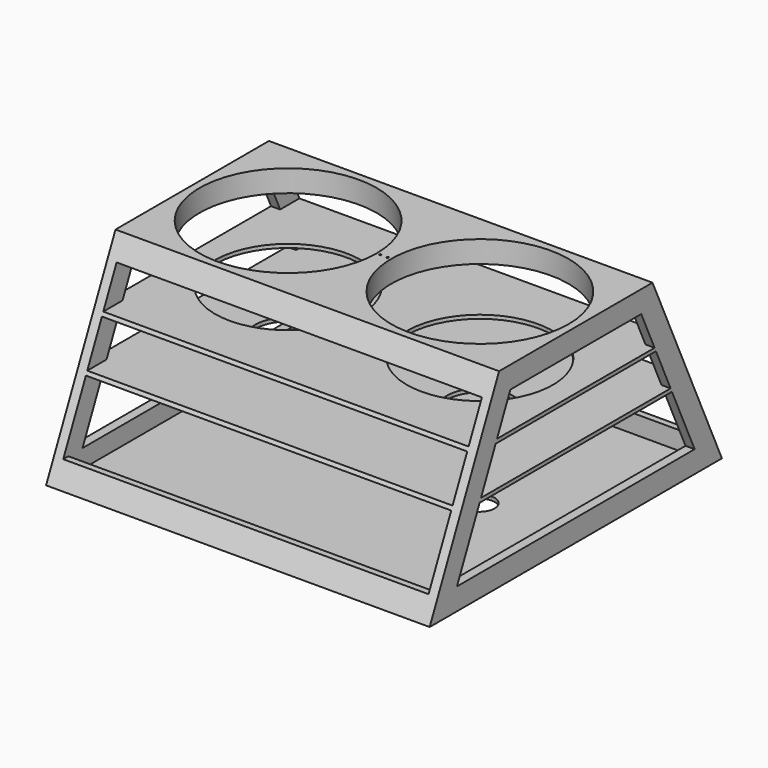
from build123d import *

# Parameters (mm, degrees)
F0_W      = 666.75
F0_H      = 635
F1_DEPTH  = 165.1
F4_W      = 333.375
F4_H      = 69.85
F5_DEPTH  = 666.751
F6_W      = 635
F6_H      = 63.5
F6_H_2    = 107.95
F6_H_3    = 69.85
F7_DEPTH  = 330.2
F9_DEPTH  = 38.1
F11_DEPTH = 25.4
F13_DEPTH = 25.4
F14_W     = 635
F14_H     = 577.849984169
F15_DEPTH = 31.75
F17_DEPTH = 25.4
F19_D     = 3.175
F19_DEPTH = 38.1
F19_TIP   = 0.9538662327


with BuildPart() as f1:
    # F0 (on Top) → F1 (new body, symmetric)
    with BuildSketch(Plane.XY):
        Rectangle(F0_W, F0_H)
    extrude(amount=F1_DEPTH, both=True)

    # F4 (on face) → F5 (cut, through all)
    with BuildSketch(Plane.YZ.offset(333.375)):
        Polygon((0, 127), (-142.2031428718, 127), (-166.6875, 73.3921443929), (-166.6875, 63.5), (166.6875, 63.5), (166.6875, 73.3921443929), (142.2031428718, 127), align=None)
        Polygon((-166.6875, 63.5), (-166.6875, 73.3921443929), (-171.2055467179, 63.5), align=None)
        Polygon((171.2055467179, 63.5), (166.6875, 73.3921443929), (166.6875, 63.5), align=None)
        Polygon((174.1057871025, 57.15), (166.6875, 57.15), (166.6875, -12.7), (206.0084313333, -12.7), align=None)
        with Locations((0, 22.225)):
            Rectangle(F4_W, F4_H)
        Polygon((-166.6875, -12.7), (-166.6875, 57.15), (-174.1057871025, 57.15), (-206.0084313333, -12.7), align=None)
        Polygon((-208.9086717179, -19.05), (-258.2127582564, -127), (-166.6875, -127), (-166.6875, -19.05), align=None)
        Polygon((-166.6875, -19.05), (-166.6875, -127), (0, -127), (166.6875, -127), (166.6875, -19.05), align=None)
        Polygon((166.6875, -19.05), (166.6875, -127), (258.2127582564, -127), (208.9086717179, -19.05), align=None)
        Polygon((317.5, 165.1), (166.6875, 165.1), (184.0889423077, 127), (213.0913461538, 63.5), (317.5, -165.1), align=None)
        Polygon((-184.0889423077, 127), (-166.6875, 165.1), (-317.5, 165.1), (-317.5, -165.1), (-213.0913461538, 63.5), align=None)
    extrude(amount=-F5_DEPTH, mode=Mode.SUBTRACT)

    # F6 (on Front) → F7 (cut, symmetric)
    with BuildSketch(Plane.XZ):
        with Locations((0, 95.25)):
            Rectangle(F6_W, F6_H)
        with Locations((0, -73.025)):
            Rectangle(F6_W, F6_H_2)
        with Locations((0, 22.225)):
            Rectangle(F6_W, F6_H_3)
    extrude(amount=F7_DEPTH, both=True, mode=Mode.SUBTRACT)

    # F3 (on face) + F8 (on face) → F9 (cut)
    with BuildSketch(Plane.XY.offset(165.1)):
        with BuildLine():
            ThreePointArc((-166.6875, 153.9875), (-320.675, 0), (-166.6875, -153.9875))
            Line((-166.6875, -153.9875), (-166.6875, 153.9875))
        make_face()
        with BuildLine():
            Line((-166.6875, 153.9875), (-166.6875, -153.9875))
            ThreePointArc((-166.6875, -153.9875), (-57.801894532, -108.885605468), (-12.7, 0))
            ThreePointArc((-12.7, 0), (-57.801894532, 108.885605468), (-166.6875, 153.9875))
        make_face()
        with BuildLine():
            ThreePointArc((166.6875, 153.9875), (12.7, 0), (166.6875, -153.9875))
            Line((166.6875, -153.9875), (166.6875, 153.9875))
        make_face()
    with BuildSketch(Plane.XY.offset(165.1)):
        with BuildLine():
            Line((166.6875, 153.9875), (166.6875, -153.9875))
            ThreePointArc((166.6875, -153.9875), (275.573105468, -108.885605468), (320.675, 0))
            ThreePointArc((320.675, 0), (275.573105468, 108.885605468), (166.6875, 153.9875))
        make_face()
    extrude(amount=-F9_DEPTH, mode=Mode.SUBTRACT)

    # F10 (on face) → F11 (cut)
    with BuildSketch(Plane.XY.offset(63.5)):
        with BuildLine():
            ThreePointArc((-166.6875, 127), (-293.6875, 0), (-166.6875, -127))
            Line((-166.6875, -127), (-166.6875, 127))
        make_face()
        with BuildLine():
            Line((-166.6875, 127), (-166.6875, -127))
            ThreePointArc((-166.6875, -127), (-76.8849387893, -89.8025612107), (-39.6875, 0))
            ThreePointArc((-39.6875, 0), (-76.8849387893, 89.8025612107), (-166.6875, 127))
        make_face()
        with BuildLine():
            ThreePointArc((166.6875, 127), (39.6875, 0), (166.6875, -127))
            Line((166.6875, -127), (166.6875, 127))
        make_face()
        with BuildLine():
            Line((166.6875, 127), (166.6875, -127))
            ThreePointArc((166.6875, -127), (256.4900612107, -89.8025612107), (293.6875, 0))
            ThreePointArc((293.6875, 0), (256.4900612107, 89.8025612107), (166.6875, 127))
        make_face()
    extrude(amount=-F11_DEPTH, mode=Mode.SUBTRACT)

    # F12 (on face) → F13 (cut)
    with BuildSketch(Plane.XY.offset(-12.7)):
        with BuildLine():
            ThreePointArc((-166.6875, 57.15), (-223.8375, 0), (-166.6875, -57.15))
            Line((-166.6875, -57.15), (-166.6875, 57.15))
        make_face()
        with BuildLine():
            Line((-166.6875, 57.15), (-166.6875, -57.15))
            ThreePointArc((-166.6875, -57.15), (-126.2763474552, -40.4111525448), (-109.5375, 0))
            ThreePointArc((-109.5375, 0), (-126.2763474552, 40.4111525448), (-166.6875, 57.15))
        make_face()
        with BuildLine():
            ThreePointArc((166.6875, 57.15), (109.5375, 0), (166.6875, -57.15))
            Line((166.6875, -57.15), (166.6875, 57.15))
        make_face()
        with BuildLine():
            Line((166.6875, 57.15), (166.6875, -57.15))
            ThreePointArc((166.6875, -57.15), (207.0986525448, -40.4111525448), (223.8375, 0))
            ThreePointArc((223.8375, 0), (207.0986525448, 40.4111525448), (166.6875, 57.15))
        make_face()
    extrude(amount=-F13_DEPTH, mode=Mode.SUBTRACT)

    # F14 (on face) → F15 (cut)
    with BuildSketch(Plane.XY.offset(-127)):
        Rectangle(F14_W, F14_H)
    extrude(amount=-F15_DEPTH, mode=Mode.SUBTRACT)

    # F16 (on face) → F17 (cut)
    with BuildSketch(Plane.XY.offset(-158.75)):
        with BuildLine():
            ThreePointArc((-166.6875, 25.4), (-192.0875, 0), (-166.6875, -25.4))
            Line((-166.6875, -25.4), (-166.6875, 25.4))
        make_face()
        with BuildLine():
            Line((-166.6875, 25.4), (-166.6875, -25.4))
            ThreePointArc((-166.6875, -25.4), (-148.7269877579, -17.9605122421), (-141.2875, 0))
            ThreePointArc((-141.2875, 0), (-148.7269877579, 17.9605122421), (-166.6875, 25.4))
        make_face()
        with BuildLine():
            Line((166.6875, 25.4), (166.6875, -25.4))
            ThreePointArc((166.6875, -25.4), (184.6480122421, -17.9605122421), (192.0875, 0))
            ThreePointArc((192.0875, 0), (184.6480122421, 17.9605122421), (166.6875, 25.4))
        make_face()
        with BuildLine():
            ThreePointArc((166.6875, 25.4), (141.2875, 0), (166.6875, -25.4))
            Line((166.6875, -25.4), (166.6875, 25.4))
        make_face()
    extrude(amount=-F17_DEPTH, mode=Mode.SUBTRACT)

    # F19
    with Locations(Plane.XY.offset(165.1)):
        with Locations((-6.35, 0), (6.35, 0)):
            Hole(F19_D / 2, depth=F19_DEPTH)
            with Locations((0, 0, -(F19_DEPTH + F19_TIP / 2))):  # 118° drill point
                Cone(0, F19_D / 2, F19_TIP, mode=Mode.SUBTRACT)


solid = f1.part
